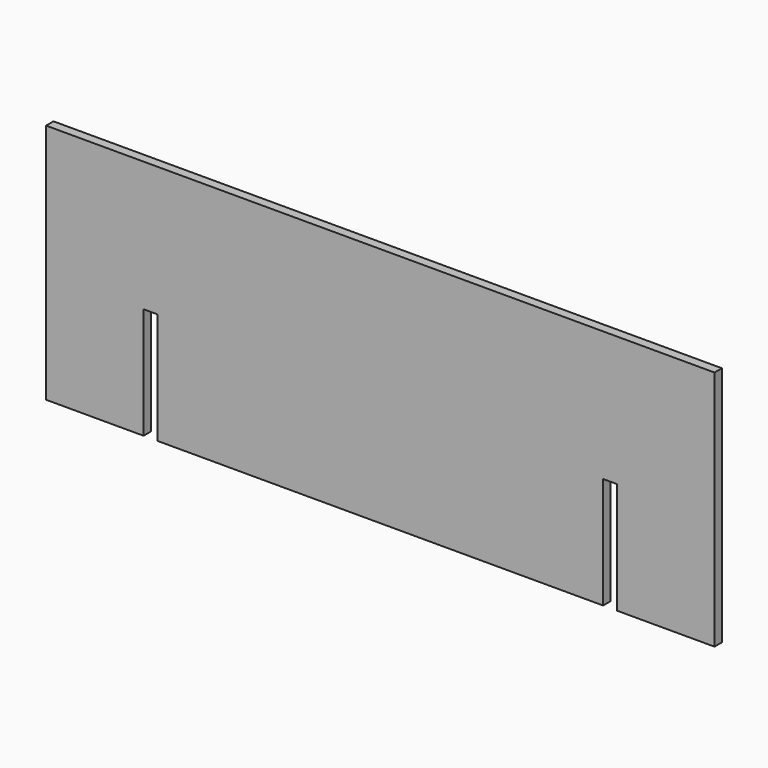
from build123d import *

# Parameters (mm, degrees)
F0_W     = 914.4
F0_H     = 330.2
F1_DEPTH = 6.35
F2_W     = 19.05
F2_H     = 152.4
F3_DEPTH = 12.701


# Not quite as in the source:
# - a pattern or mirror of a feature is missing from the dataset's text; its kind, count and spacing are read off the source's solid


with BuildPart() as f1:
    # F0 (on Front) → F1 (new body, symmetric)
    with BuildSketch(Plane.XZ):
        Rectangle(F0_W, F0_H)
    extrude(amount=F1_DEPTH, both=True)

    # F2 (on face) → F3 (cut, through all)
    with BuildSketch(Plane.XZ.offset(6.35)):
        with Locations((314.325, -88.9)):
            Rectangle(F2_W, F2_H)
    f3 = extrude(amount=-F3_DEPTH, mode=Mode.SUBTRACT)

    # F3_copies: F3 across plane
    add(f3.mirror(Plane(origin=(0, 0, 0), x_dir=(0, 0, -1), z_dir=(-1, 0, 0))), mode=Mode.SUBTRACT)


solid = f1.part
